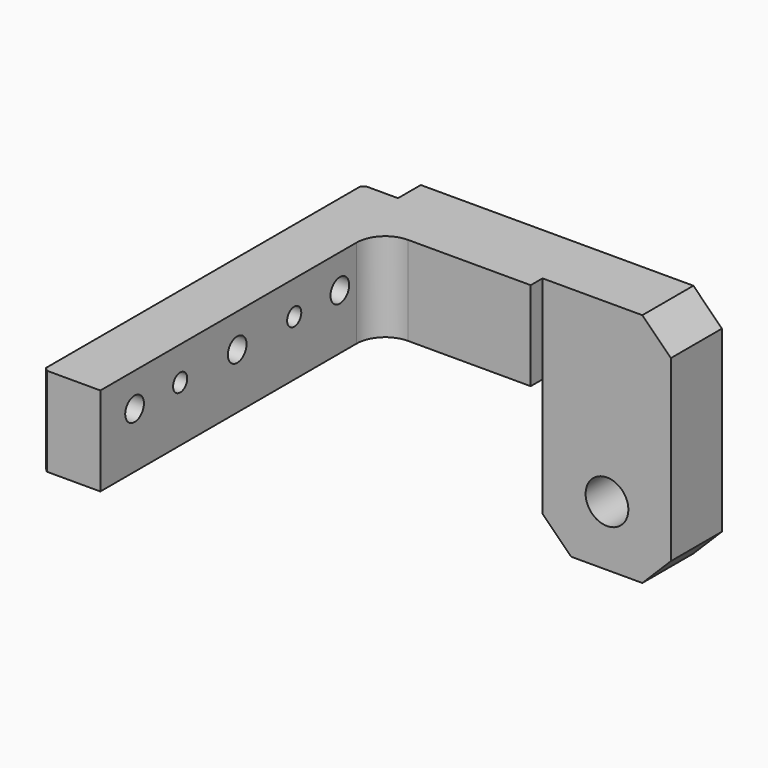
from build123d import *

# Parameters (mm, degrees)
F3_DEPTH = 14.224
F4_START = 22.352
F1_W     = 77.0001
F1_H     = 15.748
F4_DEPTH = 39.624
F5_DEPTH = 121.4511
F6_SIZE2 = 12.7
F6_SIZE  = 12.7
F7_SIZE  = 1.524


with BuildPart() as f3:
    # F0 (on Front) → F3 (new body, symmetric)
    with BuildSketch(Plane.XZ):
        Polygon((-28.702, -43.053), (28.448, -43.053), (28.448, 53.848), (-28.702, 53.848), (-28.702, 15.748), align=None)
        with BuildLine():
            ThreePointArc((-4.924195, -8.1534), (-4.680955, 8.295438), (9.525, 0))
            ThreePointArc((9.525, 0), (8.295438, -4.680955), (4.924195, -8.1534))
            ThreePointArc((4.924195, -8.1534), (8.295438, -11.625845), (9.525, -16.3068))
            ThreePointArc((9.525, -16.3068), (-4.680955, -24.602238), (-4.924195, -8.1534))
        make_face(mode=Mode.SUBTRACT)
        with BuildLine():
            ThreePointArc((4.924195, -8.1534), (8.295438, -4.680955), (9.525, 0))
            ThreePointArc((9.525, 0), (-4.680955, 8.295438), (-4.924195, -8.1534))
            ThreePointArc((-4.924195, -8.1534), (0, -6.7818), (4.924195, -8.1534))
        make_face()
    extrude(amount=F3_DEPTH, both=True)

    # F1 (on Top) → F4 (join)
    with BuildSketch(Plane.XY.offset(F4_START)):
        Polygon((-28.702, -14.224), (28.448, -14.224), (28.448, 14.224), (-105.7021, 14.224), (-105.7021, 1.524), (-28.702, 1.524), align=None)
        with Locations((-67.20205, -6.35)):
            Rectangle(F1_W, F1_H)
        Polygon((-28.702, -20.828), (-28.702, -14.224), (-105.7021, -14.224), (-105.7021, 1.524), (-121.4501, 1.524), (-121.4501, -20.828), (-96.0501, -20.828), (-83.3501, -20.828), align=None)
        Polygon((-96.0501, -33.528), (-96.0501, -20.828), (-121.4501, -20.828), (-121.4501, -176.276), (-96.0501, -176.276), align=None)
        with BuildLine():
            ThreePointArc((-96.0501, -33.528), (-92.330356, -24.547744), (-83.3501, -20.828))
            Line((-83.3501, -20.828), (-96.0501, -20.828))
            Line((-96.0501, -20.828), (-96.0501, -33.528))
        make_face()
    extrude(amount=F4_DEPTH)

    # F2 (on Right) → F5 (cut, through all)
    with BuildSketch(Plane.YZ):
        with BuildLine():
            ThreePointArc((-48.133, 47.0408), (-42.926, 41.8338), (-37.719, 47.0408))
            Line((-37.719, 47.0408), (-48.133, 47.0408))
        make_face()
        with BuildLine():
            Line((-48.133, 47.0408), (-37.719, 47.0408))
            ThreePointArc((-37.719, 47.0408), (-42.926, 52.2478), (-48.133, 47.0408))
        make_face()
        with BuildLine():
            ThreePointArc((-72.263, 47.0408), (-68.326, 43.1038), (-64.389, 47.0408))
            Line((-64.389, 47.0408), (-72.263, 47.0408))
        make_face()
        with BuildLine():
            Line((-72.263, 47.0408), (-64.389, 47.0408))
            ThreePointArc((-64.389, 47.0408), (-68.326, 50.9778), (-72.263, 47.0408))
        make_face()
        with BuildLine():
            ThreePointArc((-105.283, 47.0408), (-100.076, 41.8338), (-94.869, 47.0408))
            Line((-94.869, 47.0408), (-105.283, 47.0408))
        make_face()
        with BuildLine():
            Line((-105.283, 47.0408), (-94.869, 47.0408))
            ThreePointArc((-94.869, 47.0408), (-100.076, 52.2478), (-105.283, 47.0408))
        make_face()
        with BuildLine():
            Line((-127.889, 47.0408), (-135.763, 47.0408))
            ThreePointArc((-135.763, 47.0408), (-131.826, 43.1038), (-127.889, 47.0408))
        make_face()
        with BuildLine():
            ThreePointArc((-127.889, 47.0408), (-131.826, 50.9778), (-135.763, 47.0408))
            Line((-135.763, 47.0408), (-127.889, 47.0408))
        make_face()
        with BuildLine():
            Line((-152.019, 47.0408), (-162.433, 47.0408))
            ThreePointArc((-162.433, 47.0408), (-157.226, 41.8338), (-152.019, 47.0408))
        make_face()
        with BuildLine():
            ThreePointArc((-152.019, 47.0408), (-157.226, 52.2478), (-162.433, 47.0408))
            Line((-162.433, 47.0408), (-152.019, 47.0408))
        make_face()
    extrude(amount=-F5_DEPTH, mode=Mode.SUBTRACT)

    # F6
    f6_edges = [f3.edges().sort_by_distance(p)[0] for p in [
        (28.448, 0, -43.053),
        (-28.702, 0, -43.053),
        (28.448, 0, 61.976),
    ]]
    chamfer(f6_edges, length=F6_SIZE, length2=F6_SIZE2)

    # F7
    f7_edges = [f3.edges().sort_by_distance(p)[0] for p in [
        (-121.4501, -176.276, 42.164),
        (-121.4501, 1.524, 42.164),
    ]]
    chamfer(f7_edges, length=F7_SIZE)


solid = f3.part
